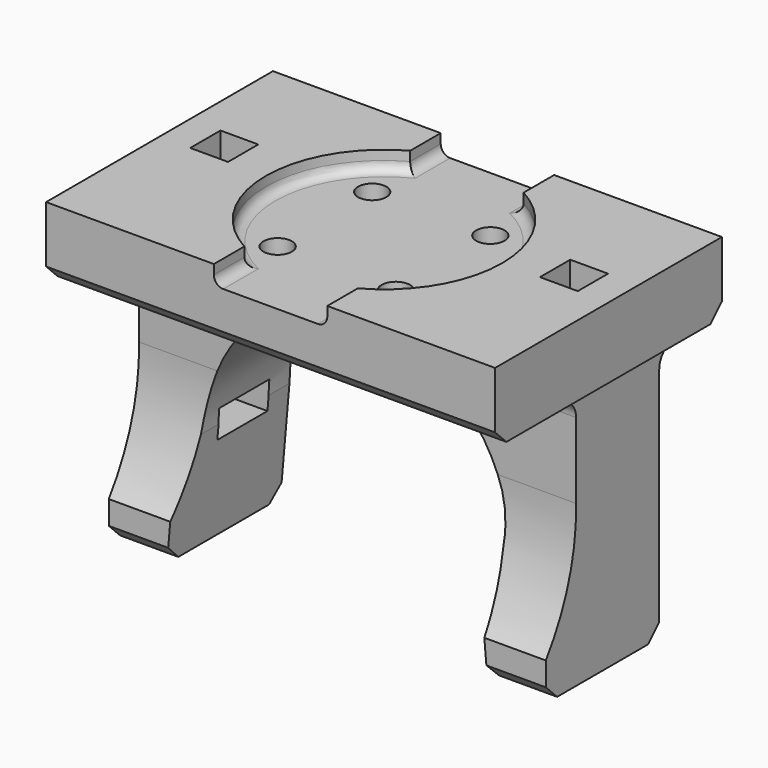
from build123d import *

# Parameters (mm, degrees)
F0_W      = 95
F0_H      = 60
F1_DEPTH  = 15
F3_DEPTH  = 15
F5_W      = 13.25
F5_H      = 6.05
F6_DEPTH  = 10
F7_W      = 8
F7_H      = 8
F8_DEPTH  = 29
F11_DEPTH = 93
F12_SIZE  = 3
F14_DEPTH = 4
F15_R     = 3
F16_DEPTH = 6
F17_R     = 2
F18_R     = 4


with BuildPart() as f1:
    # F0 (on Top) → F1 (new body)
    with BuildSketch(Plane.XY):
        Rectangle(F0_W, F0_H)
    extrude(amount=F1_DEPTH)

    # F2 (on Front) → F3 (join, symmetric)
    with BuildSketch(Plane.XZ):
        with BuildLine():
            Line((-3.075, 0), (-46.235655491, 0))
            Line((-46.235655491, 0), (-46.235655491, -54))
            Line((-46.235655491, -54), (-33.9247505976, -54))
            Line((-33.9247505976, -54), (-32, -32))
            ThreePointArc((-32, -32), (-23.6896601917, -10.4872131048), (-3.075, -0.1480867922))
            Line((-3.075, -0.1480867922), (-3.075, 0))
        make_face()
        with BuildLine():
            Line((3.075, 0), (3.075, -0.1480867922))
            ThreePointArc((3.075, -0.1480867922), (23.6896601917, -10.4872131048), (32, -32))
            Line((32, -32), (33.9247505976, -54))
            Line((33.9247505976, -54), (46.235655491, -54))
            Line((46.235655491, -54), (46.235655491, 0))
            Line((46.235655491, 0), (3.075, 0))
        make_face()
    extrude(amount=F3_DEPTH, both=True)

    # F5 (on offset) → F6 (cut, symmetric)
    with BuildSketch(Plane.YZ.offset(-32)):
        with Locations((2.875, -32)):
            Rectangle(F5_W, F5_H)
    extrude(amount=F6_DEPTH, both=True, mode=Mode.SUBTRACT)

    # F7 (on Top) → F8 (cut, symmetric)
    with BuildSketch(Plane.XY):
        with Locations((-37, 4)):
            Rectangle(F7_W, F7_H)
    extrude(amount=F8_DEPTH, both=True, mode=Mode.SUBTRACT)

    # F9: F1 across plane


with BuildPart() as f1_1:
    add(f1.part)
    add(f1.part.mirror(Plane.YZ), mode=Mode.INTERSECT)

    # F10 (on face) → F11 (cut)
    with BuildSketch(Plane.YZ.offset(46.235655491)):
        with BuildLine():
            Line((-7, -20), (-7, 0))
            Line((-7, 0), (-15, 0))
            Line((-15, 0), (-15, -46))
            ThreePointArc((-15, -46), (-8.8897891542, -33.6492956449), (-7, -20))
        make_face()
    extrude(amount=-F11_DEPTH, mode=Mode.SUBTRACT)

    # F12
    f12_edges = [f1_1.edges().sort_by_distance(p)[0] for p in [
        (40.080203, -15, -54),
        (-40.080203, -15, -54),
        (0, -30, 0),
        (0, 30, 0),
        (40.080203, 15, -54),
        (-40.080203, 15, -54),
    ]]
    chamfer(f12_edges, length=F12_SIZE)

    # F13 (on face) → F14 (cut)
    with BuildSketch(Plane.XY.offset(15)):
        with BuildLine():
            Line((-12, 30), (-12, 21.9317121995))
            ThreePointArc((-12, 21.9317121995), (-25, 0), (-12, -21.9317121995))
            Line((-12, -21.9317121995), (-12, -30))
            Line((-12, -30), (12, -30))
            Line((12, -30), (12, -21.9317121995))
            ThreePointArc((12, -21.9317121995), (25, 0), (12, 21.9317121995))
            Line((12, 21.9317121995), (12, 30))
            Line((12, 30), (-12, 30))
        make_face()
    extrude(amount=-F14_DEPTH, mode=Mode.SUBTRACT)

    # F15 (on face) → F16 (cut)
    with BuildSketch(Plane.XY.offset(11)):
        with Locations((12.5, -12.5)):
            Circle(F15_R)
        with Locations((-12.5, -12.5)):
            Circle(F15_R)
        with Locations((-12.5, 12.5)):
            Circle(F15_R)
        with Locations((12.5, 12.5)):
            Circle(F15_R)
    extrude(amount=-F16_DEPTH, mode=Mode.SUBTRACT)

    # F17
    f17_edges = [f1_1.edges().sort_by_distance(p)[0] for p in [
        (-25, 0, 11),
        (25, 0, 11),
        (-12, -25.965856, 11),
        (12, -25.965856, 11),
        (12, 25.965856, 11),
        (-12, 25.965856, 11),
    ]]
    fillet(f17_edges, radius=F17_R)

    # F18 (call 1 of 4: OpenCascade refuses the feature's edges together)
    f18_edges = [f1_1.edges().sort_by_distance(p)[0] for p in [
        (-24.655328, -7, 0),
    ]]
    fillet(f18_edges, radius=F18_R)

    # F18#2 (call 2 of 4)
    f18_2_edges = [f1_1.edges().sort_by_distance(p)[0] for p in [
        (24.655328, -7, 0),
    ]]
    fillet(f18_2_edges, radius=F18_R)

    # F18#3 (call 3 of 4)
    f18_3_edges = [f1_1.edges().sort_by_distance(p)[0] for p in [
        (24.655328, 15, 0),
    ]]
    fillet(f18_3_edges, radius=F18_R)

    # F18#4 (call 4 of 4)
    f18_4_edges = [f1_1.edges().sort_by_distance(p)[0] for p in [
        (-24.655328, 15, 0),
    ]]
    fillet(f18_4_edges, radius=F18_R)


solid = f1_1.part
